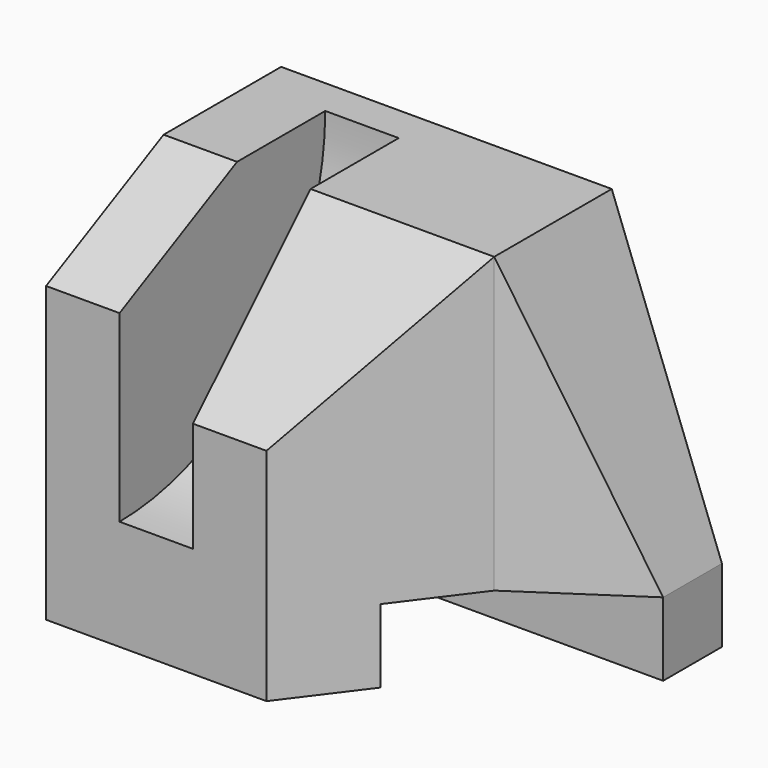
from build123d import *

# Parameters (mm, degrees)
F0_W      = 60
F0_H      = 40
F1_DEPTH  = 50
F2_W      = 10
F2_H      = 35
F3_DEPTH  = 35
F4_R      = 34.99999
F5_W      = 20
F5_H      = 10
F6_DEPTH  = 60.001
F8_DEPTH  = 50.001
F10_DEPTH = 50.001
F17_W     = 10
F17_H     = 20


# Not quite as in the source:
# - a fillet or chamfer is up to 0.001 mm smaller than in the source, because OpenCascade refuses the exact size


with BuildPart() as f1:
    # F0 (on Top) → F1 (new body)
    with BuildSketch(Plane.XY):
        with Locations((30, 20)):
            Rectangle(F0_W, F0_H)
    extrude(amount=F1_DEPTH)

    # F2 (on face) → F3 (cut)
    with BuildSketch(Plane.XY.offset(50)):
        with Locations((15, 17.5)):
            Rectangle(F2_W, F2_H)
    extrude(amount=-F3_DEPTH, mode=Mode.SUBTRACT)

    # F4 (radius 35 in the source; OpenCascade refuses exactly that, so slightly less here)
    f4_edges = [f1.edges().sort_by_distance(p)[0] for p in [
        (15, 35, 15),
    ]]
    fillet(f4_edges, radius=F4_R)

    # F5 (on face) → F6 (cut, through all)
    with BuildSketch(Plane.YZ.offset(60)):
        with Locations((20, 5)):
            Rectangle(F5_W, F5_H)
    extrude(amount=-F6_DEPTH, mode=Mode.SUBTRACT)

    # F7 (on face) → F8 (cut, through all)
    with BuildSketch(Plane.XY.offset(50)):
        Polygon((45, 20), (60, 20), (60, 30), align=None)
    extrude(amount=-F8_DEPTH, mode=Mode.SUBTRACT)

    # F9 (on face) → F10 (cut, through all)
    with BuildSketch(Plane.XY.offset(50)):
        Polygon((60, 20), (45, 20), (30, 0), (60, 0), align=None)
    extrude(amount=-F10_DEPTH, mode=Mode.SUBTRACT)

    # F13: sweep along a path in F12
    with BuildLine(Plane(origin=(0, 40, 0), x_dir=(-1, 0, 0), z_dir=(0, 1, 0))) as f13_path:
        Line((-45, 50), (-60, 10))
    # F11 (on face) → F13 (sweep, cut)
    with BuildSketch(Plane.XY.offset(50)):
        Polygon((45, 40), (45, 20), (60, 30), (60, 40), align=None)
    sweep(path=f13_path.line, mode=Mode.SUBTRACT)

    # F16: sweep along a path in F15
    with BuildLine(Plane(origin=(20, 0, 0), x_dir=(0, -1, 0), z_dir=(-1, 0, 0))) as f16_path:
        Line((-20, 50), (0, 30))
    # F14 (on face) → F16 (sweep, cut)
    with BuildSketch(Plane.XY.offset(50)):
        Polygon((30, 0), (45, 20), (20, 20), (20, 0), align=None)
    sweep(path=f16_path.line, mode=Mode.SUBTRACT)

    # F19: sweep along a path in F18
    with BuildLine(Plane(origin=(0, 0, 0), x_dir=(0, -1, 0), z_dir=(-1, 0, 0))) as f19_path:
        Line((-20, 50), (0, 40))
    # F17 (on face) → F19 (sweep, cut)
    with BuildSketch(Plane.XY.offset(50)):
        with Locations((5, 10)):
            Rectangle(F17_W, F17_H)
    sweep(path=f19_path.line, mode=Mode.SUBTRACT)


solid = f1.part
